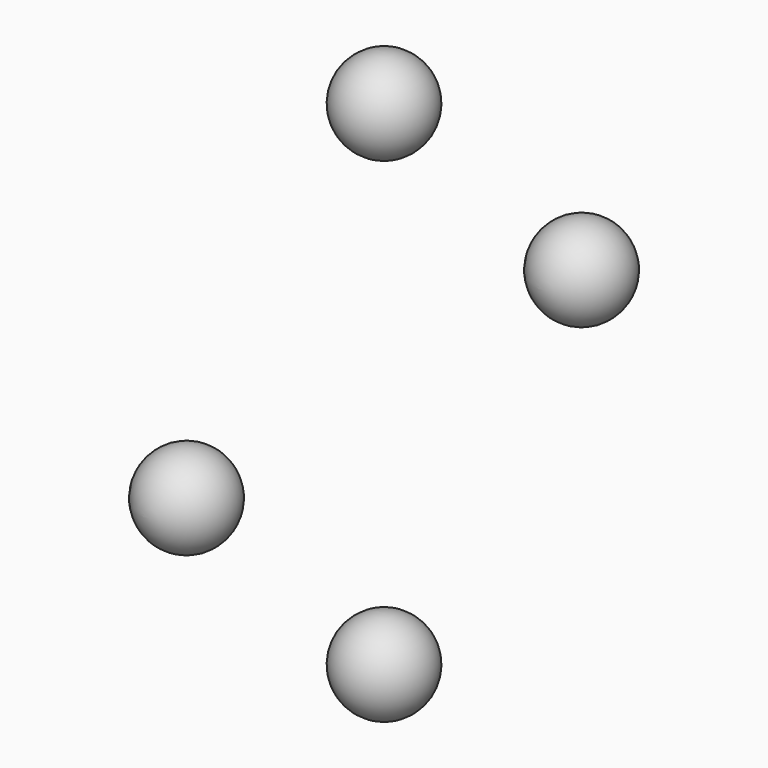
from build123d import *

# Parameters (mm, degrees)
F1_COPIES_COUNT = 4


# Not quite as in the source:
# - a pattern or mirror of a feature is missing from the dataset's text; its kind, count and spacing are read off the source's solid


with BuildPart() as f1:
    # F0 (on Front) → F1 (revolve)
    with BuildSketch(Plane.XZ):
        with BuildLine():
            Line((0, 22.5), (0, 32.5))
            ThreePointArc((0, 32.5), (-5, 27.5), (0, 22.5))
        make_face()
    revolve(axis=Axis((0, 0, 27.5), (0, 0, -1)))


with BuildPart() as f1_copies_1:
    # F1_copies: instance of F1
    add(f1.part.rotate(Axis((0, 0, 0), (1, 0, 0)), 1 * 360 / F1_COPIES_COUNT))


with BuildPart() as f1_copies_2:
    # F1_copies: instance of F1
    add(f1.part.rotate(Axis((0, 0, 0), (1, 0, 0)), 2 * 360 / F1_COPIES_COUNT))


with BuildPart() as f1_copies_3:
    # F1_copies: instance of F1
    add(f1.part.rotate(Axis((0, 0, 0), (1, 0, 0)), 3 * 360 / F1_COPIES_COUNT))


solid = Compound([f1.part, f1_copies_1.part, f1_copies_2.part, f1_copies_3.part])
